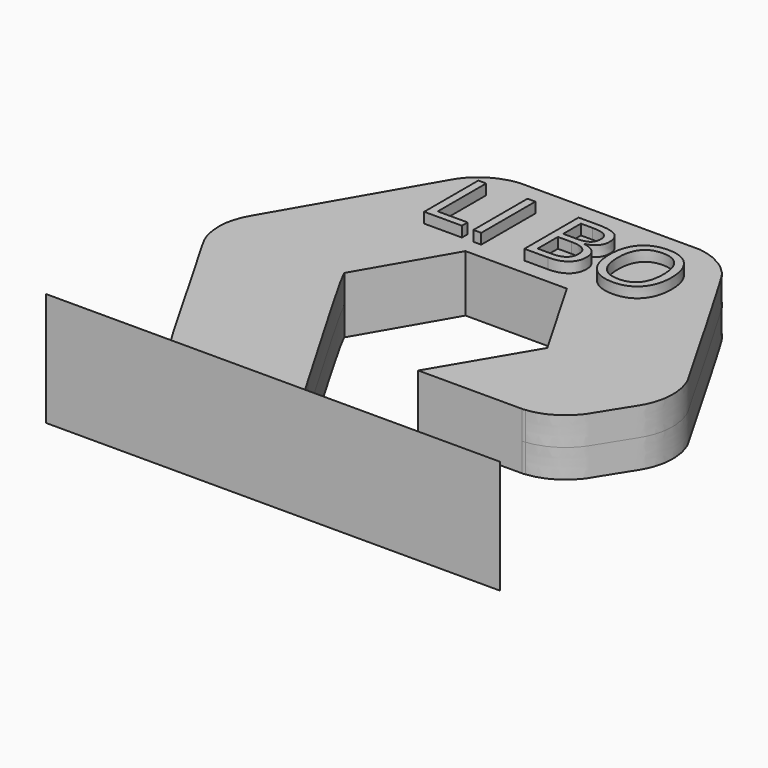
from build123d import *

# Parameters (mm, degrees)
F1_DEPTH     = 3.175
F2_DEPTH     = 1.5875
F3_DEPTH     = 1.5875
F4_T1_DEPTH  = 22.6801869736
F4_T3_DEPTH  = 41.7253830583
F5_TEXT_SIZE = 5.3007951162
F6_DEPTH     = 0.5842


# Not quite as in the source:
# - a fillet or chamfer that OpenCascade refuses, or shapes differently, is made with other operations: its cross-section is extruded or revolved along the edge and cut away or added
# - Text() gives the source's letters only with a copy of the font that has no kerning and outlines rounded to 1/6400 em; it was checked with that copy


with BuildPart() as f1:
    # F0 (on Top) → F1 (new body, symmetric)
    with BuildSketch(Plane.XY):
        with BuildLine():
            add(Edge.make_bspline(
                [(-8.0979492671, -8.4599665572), (-7.8144543772, -8.9512922446), (-7.4012331652, -9.6478596679), (-7.2094447017, -9.853233929), (-7.0198074368, -10.0624663427), (-6.8247908118, -10.2363901293), (-6.6355575508, -10.3900701529), (-6.4438841868, -10.5234739102), (-6.0350828964, -10.7264789939), (-5.8763022274, -10.78836422), (-5.4940772788, -10.9232334645), (-5.1611591338, -10.9716922009), (-4.9454318311, -10.9894729499), (-4.8368193396, -10.9980083466), (-1.8185705834, -10.9990381649), (0.9024133324, -10.9999665572)],
                knots=[0.5399683447, 0.5399683447, 0.5399683447, 0.5399683447, 0.583735527, 0.615598334, 0.6417416026, 0.6683965868, 0.6934366825, 0.7191935337, 0.7535274628, 0.7758085206, 0.8081226598, 0.8394404995, 0.861841058, 0.8754482187, 1, 1, 1, 1], degree=3))
            Line((-8.0979492671, -8.4599665572), (-12.7, -8.4599665572))
            Line((-12.7, -8.4599665572), (-12.7, -11.6349665572))
            Line((-12.7, -11.6349665572), (12.6951960847, -11.6349665572))
            Line((12.6951960847, -11.6349665572), (12.6951960847, -8.4599665572))
            Line((12.6951960847, -8.4599665572), (-0.5820742577, -8.4599665572))
            add(Edge.make_bspline(
                [(-0.5820742577, -8.4599665572), (-0.0948763272, -9.2939885426), (0.4037685026, -10.1469775499), (0.9024133324, -10.9999665572)],
                knots=[0.8523529488, 0.8523529488, 0.8523529488, 0.8523529488, 1, 1, 1, 1], degree=3))
        make_face()
        with BuildLine():
            Line((-0.5820742577, -8.4599665572), (-8.0979492671, -8.4599665572))
            add(Edge.make_bspline(
                [(-8.0979492671, -8.4599665572), (-7.8144543772, -8.9512922446), (-7.4012331652, -9.6478596679), (-7.2094447017, -9.853233929), (-7.0198074368, -10.0624663427), (-6.8247908118, -10.2363901293), (-6.6355575508, -10.3900701529), (-6.4438841868, -10.5234739102), (-6.0350828964, -10.7264789939), (-5.8763022274, -10.78836422), (-5.4940772788, -10.9232334645), (-5.1611591338, -10.9716922009), (-4.9454318311, -10.9894729499), (-4.8368193396, -10.9980083466), (-1.8185705834, -10.9990381649), (0.9024133324, -10.9999665572)],
                knots=[0.5399683447, 0.5399683447, 0.5399683447, 0.5399683447, 0.583735527, 0.615598334, 0.6417416026, 0.6683965868, 0.6934366825, 0.7191935337, 0.7535274628, 0.7758085206, 0.8081226598, 0.8394404995, 0.861841058, 0.8754482187, 1, 1, 1, 1], degree=3))
            add(Edge.make_bspline(
                [(-0.5820742577, -8.4599665572), (-0.0948763272, -9.2939885426), (0.4037685026, -10.1469775499), (0.9024133324, -10.9999665572)],
                knots=[0.8523529488, 0.8523529488, 0.8523529488, 0.8523529488, 1, 1, 1, 1], degree=3))
        make_face()
    extrude(amount=F1_DEPTH, both=True)

    # F0 (on Top) → F2 (cut, symmetric)
    with BuildSketch(Plane.XY):
        with BuildLine():
            add(Edge.make_bspline(
                [(-4.9467352219, 11.8727972619), (-2.6941970372, 11.8727972619), (-0.4416588525, 11.8727972619), (1.8108793323, 11.8727972619)],
                knots=[0.5524163134, 0.5524163134, 0.5524163134, 0.5524163134, 7.3100308676, 7.3100308676, 7.3100308676, 7.3100308676], degree=3))
            add(Edge.make_bspline(
                [(-12.1819954365, 2.2322773002), (-10.2153621206, 5.6292283823), (-7.918654142, 9.5963149713), (-7.7561059918, 9.8938723276), (-7.595936966, 10.1748103574), (-7.4488921306, 10.429639936), (-7.2380091716, 10.7143793357), (-7.0022497381, 10.9732635429), (-6.7468930063, 11.1814042046), (-6.6123462397, 11.2802086076), (-6.44534623, 11.390971666), (-6.3180815613, 11.463666659), (-6.1526142879, 11.5500745414), (-6.0434056072, 11.6051608595), (-5.8991320293, 11.660363592), (-5.6381957934, 11.7542790581), (-5.4211920209, 11.8110346891), (-5.1249038455, 11.8530818861), (-5.1009011539, 11.8676549492), (-4.9467352219, 11.8727972619)],
                knots=[0, 0, 0, 0, 0.1520022985, 0.1775139721, 0.2052814017, 0.2338919375, 0.2644870562, 0.2956347735, 0.3249719317, 0.3463123249, 0.3689682109, 0.3892301717, 0.411329997, 0.4293235674, 0.449497138, 0.4765503291, 0.5022012755, 0.5278147587, 0.5520405652, 0.5520405652, 0.5520405652, 0.5520405652], degree=3))
            add(Edge.make_bspline(
                [(-12.1819954365, 2.2322773002), (-12.2139037883, 2.1703194424), (-12.283482926, 2.0352145533), (-12.4406884255, 1.7801306072), (-12.6198918883, 1.2441500466), (-12.7164267868, 0.7551726738), (-12.7062312963, 0.3123164438), (-12.6510102494, -0.2863243011), (-12.5128439568, -0.6906531958), (-12.348735221, -1.0976190794), (-11.6470462247, -2.2552827891), (-11.0471565611, -3.3365181876), (-9.6670924889, -5.6885534643), (-8.4674528036, -7.819579074), (-8.0979492671, -8.4599665572)],
                knots=[0, 0, 0, 0, 0.0239021006, 0.0521207603, 0.0910959498, 0.1277402468, 0.1623042864, 0.2023672629, 0.23552051, 0.2695660314, 0.3281617082, 0.3861383143, 0.4829227709, 0.5399683447, 0.5399683447, 0.5399683447, 0.5399683447], degree=3))
            Line((-8.0979492671, -8.4599665572), (-0.5820742577, -8.4599665572))
            add(Edge.make_bspline(
                [(-5.6781647727, 0.4474149318), (-5.6798237666, 0.4432516249), (-5.716895521, 0.3502186819), (-3.2687593621, -3.8606973389), (-0.5820742577, -8.4599665572)],
                knots=[0, 0, 0, 0, 0.0381435521, 0.8523529488, 0.8523529488, 0.8523529488, 0.8523529488], degree=3))
            add(Edge.make_bspline(
                [(-2.836742904, 5.3628673777), (-3.7838835269, 3.7243832291), (-4.7310241498, 2.0858990805), (-5.6781647727, 0.4474149318)],
                knots=[0, 0, 0, 0, 5.6776184253, 5.6776184253, 5.6776184253, 5.6776184253], degree=3))
            add(Edge.make_bspline(
                [(2.8362337034, 5.3595150821), (0.9452415009, 5.360632514), (-0.9457507016, 5.3617499458), (-2.836742904, 5.3628673777)],
                knots=[0, 0, 0, 0, 5.6729775979, 5.6729775979, 5.6729775979, 5.6729775979], degree=3))
            add(Edge.make_bspline(
                [(5.6763379835, 0.4443899379), (4.7296365568, 2.082764986), (3.7829351301, 3.721140034), (2.8362337034, 5.3595150821)],
                knots=[0, 0, 0, 0, 5.6766757442, 5.6766757442, 5.6766757442, 5.6766757442], degree=3))
            add(Edge.make_bspline(
                [(2.6081528049, -4.7463672236), (3.6308811978, -3.0161148364), (4.6536095906, -1.2858624492), (5.6763379835, 0.4443899379)],
                knots=[0, 0, 0, 0, 6.0297363292, 6.0297363292, 6.0297363292, 6.0297363292], degree=3))
            Line((2.6081528049, -4.7463672236), (8.3983913064, -4.7463672236))
            add(Edge.make_bspline(
                [(8.3983913064, -4.7463672236), (8.4285802649, -4.7476342502), (8.4896773359, -4.7501984863), (8.5516653278, -4.7371940519), (8.5830241442, -4.7306152992)],
                knots=[0, 0, 0, 0, 0.4941146609, 1, 1, 1, 1], degree=3))
            add(Edge.make_bspline(
                [(7.394594606, 10.4755461216), (7.4049946498, 10.4644086633), (7.4978359113, 10.3649844979), (12.37583426, 1.9246802289), (12.3732313137, 1.8788009391), (12.4554314204, 1.7100351498), (12.5092309984, 1.5407375676), (12.579223391, 1.3481749221), (12.6327811924, 1.1548508933), (12.6617328431, 0.9474132467), (12.6887145756, 0.7331187902), (12.7057320419, 0.4773166934), (12.6885501549, 0.1892988959), (12.6579644324, -0.1503660031), (12.6047454763, -0.3551130001), (12.5476882015, -0.5689364186), (12.4644072913, -0.7996513773), (12.3592844301, -1.0395808564), (12.2025247276, -1.3122675142), (11.5798542764, -2.2842021351), (11.0022863487, -3.2119016224), (10.8931559285, -3.3988812592), (10.7117863794, -3.6224692911), (10.497630846, -3.8442513774), (10.2817003921, -4.0291717223), (10.0560553294, -4.2067210739), (9.8433649464, -4.3187164368), (9.7865197525, -4.3546553415), (9.5130416542, -4.505924573), (9.2077822138, -4.5905623978), (9.0144989656, -4.6706733119), (8.6495598585, -4.7218623963), (8.5981329416, -4.7286277074), (8.5830241442, -4.7306152992)],
                knots=[0, 0, 0, 0, 0.0211617068, 0.1889107002, 0.2086954298, 0.2296465529, 0.2530764843, 0.2773859957, 0.3015816681, 0.3261482383, 0.3512044462, 0.3783001026, 0.40768826, 0.4390979831, 0.4639315394, 0.4889953709, 0.5158573886, 0.5426802508, 0.5721507083, 0.6312181763, 0.6877344447, 0.7121562897, 0.7402266081, 0.7704940169, 0.7992541414, 0.828820597, 0.8543275782, 0.8684516809, 0.8979328023, 0.9286239977, 0.9544581079, 0.9866201736, 1, 1, 1, 1], degree=3))
            add(Edge.make_bspline(
                [(5.0841737539, 11.8727972619), (5.1354007842, 11.8660248609), (5.285102127, 11.8344246259), (5.511192311, 11.7972110307), (5.856974007, 11.6822825291), (6.0571511062, 11.6028524692), (6.5572225021, 11.3301125557), (6.8102335511, 11.1329565648), (7.0714115659, 10.8810767284), (7.2647332021, 10.6836819238), (7.3523685742, 10.5432240362), (7.394594606, 10.4755461216)],
                knots=[0.7441231562, 0.7441231562, 0.7441231562, 0.7441231562, 0.7668331465, 0.7924407066, 0.8229285687, 0.8479598314, 0.8863005426, 0.9166541286, 0.9473218688, 0.974617687, 1, 1, 1, 1], degree=3))
            add(Edge.make_bspline(
                [(4.7206622548, 11.8727972619), (4.8418327545, 11.8727972619), (4.9630032542, 11.8727972619), (5.0841737539, 11.8727972619)],
                knots=[10.2198137902, 10.2198137902, 10.2198137902, 10.2198137902, 10.5833252892, 10.5833252892, 10.5833252892, 10.5833252892], degree=3))
            add(Edge.make_bspline(
                [(1.8108793323, 11.8727972619), (3.1458171486, 11.8689304093), (4.2714307431, 11.8669693291), (4.7206622548, 11.8727972619)],
                knots=[0.6587883417, 0.6587883417, 0.6587883417, 0.6587883417, 0.7129256384, 0.7129256384, 0.7129256384, 0.7129256384], degree=3))
        make_face()
        with BuildLine():
            Line((-0.5820742577, -8.4599665572), (-8.0979492671, -8.4599665572))
            add(Edge.make_bspline(
                [(-8.0979492671, -8.4599665572), (-7.8144543772, -8.9512922446), (-7.4012331652, -9.6478596679), (-7.2094447017, -9.853233929), (-7.0198074368, -10.0624663427), (-6.8247908118, -10.2363901293), (-6.6355575508, -10.3900701529), (-6.4438841868, -10.5234739102), (-6.0350828964, -10.7264789939), (-5.8763022274, -10.78836422), (-5.4940772788, -10.9232334645), (-5.1611591338, -10.9716922009), (-4.9454318311, -10.9894729499), (-4.8368193396, -10.9980083466), (-1.8185705834, -10.9990381649), (0.9024133324, -10.9999665572)],
                knots=[0.5399683447, 0.5399683447, 0.5399683447, 0.5399683447, 0.583735527, 0.615598334, 0.6417416026, 0.6683965868, 0.6934366825, 0.7191935337, 0.7535274628, 0.7758085206, 0.8081226598, 0.8394404995, 0.861841058, 0.8754482187, 1, 1, 1, 1], degree=3))
            add(Edge.make_bspline(
                [(-0.5820742577, -8.4599665572), (-0.0948763272, -9.2939885426), (0.4037685026, -10.1469775499), (0.9024133324, -10.9999665572)],
                knots=[0.8523529488, 0.8523529488, 0.8523529488, 0.8523529488, 1, 1, 1, 1], degree=3))
        make_face()
    extrude(amount=F2_DEPTH, both=True, mode=Mode.SUBTRACT)

    # F4: chamfer of 3.175 on 4 edges, made by hand

    # F4_s2 → F4_t1 (cut)
    with BuildSketch(Plane.XY.offset(-11.3400934868)):
        Polygon((-9.525, -8.4599665572), (-12.7, -11.6349665572), (-12.7, -8.4599665572), align=None)
        Polygon((9.5201960847, -8.4599665572), (12.6951960847, -11.6349665572), (12.6951960847, -8.4599665572), align=None)
    extrude(amount=F4_T1_DEPTH, mode=Mode.SUBTRACT)

    # F4_s4 → F4_t3 (cut)
    with BuildSketch(Plane.YZ.offset(-20.8650934868)):
        Polygon((-8.4599665572, 0), (-11.6349665572, 3.175), (-8.4599665572, 3.175), align=None)
        Polygon((-8.4599665572, 0), (-11.6349665572, -3.175), (-8.4599665572, -3.175), align=None)
    extrude(amount=F4_T3_DEPTH, mode=Mode.SUBTRACT)


with BuildPart() as f3:
    # F0 (on Top) → F3 (new body, symmetric)
    with BuildSketch(Plane.XY):
        with BuildLine():
            add(Edge.make_bspline(
                [(-4.9467352219, 11.8727972619), (-2.6941970372, 11.8727972619), (-0.4416588525, 11.8727972619), (1.8108793323, 11.8727972619)],
                knots=[0.5524163134, 0.5524163134, 0.5524163134, 0.5524163134, 7.3100308676, 7.3100308676, 7.3100308676, 7.3100308676], degree=3))
            add(Edge.make_bspline(
                [(-12.1819954365, 2.2322773002), (-10.2153621206, 5.6292283823), (-7.918654142, 9.5963149713), (-7.7561059918, 9.8938723276), (-7.595936966, 10.1748103574), (-7.4488921306, 10.429639936), (-7.2380091716, 10.7143793357), (-7.0022497381, 10.9732635429), (-6.7468930063, 11.1814042046), (-6.6123462397, 11.2802086076), (-6.44534623, 11.390971666), (-6.3180815613, 11.463666659), (-6.1526142879, 11.5500745414), (-6.0434056072, 11.6051608595), (-5.8991320293, 11.660363592), (-5.6381957934, 11.7542790581), (-5.4211920209, 11.8110346891), (-5.1249038455, 11.8530818861), (-5.1009011539, 11.8676549492), (-4.9467352219, 11.8727972619)],
                knots=[0, 0, 0, 0, 0.1520022985, 0.1775139721, 0.2052814017, 0.2338919375, 0.2644870562, 0.2956347735, 0.3249719317, 0.3463123249, 0.3689682109, 0.3892301717, 0.411329997, 0.4293235674, 0.449497138, 0.4765503291, 0.5022012755, 0.5278147587, 0.5520405652, 0.5520405652, 0.5520405652, 0.5520405652], degree=3))
            add(Edge.make_bspline(
                [(-12.1819954365, 2.2322773002), (-12.2139037883, 2.1703194424), (-12.283482926, 2.0352145533), (-12.4406884255, 1.7801306072), (-12.6198918883, 1.2441500466), (-12.7164267868, 0.7551726738), (-12.7062312963, 0.3123164438), (-12.6510102494, -0.2863243011), (-12.5128439568, -0.6906531958), (-12.348735221, -1.0976190794), (-11.6470462247, -2.2552827891), (-11.0471565611, -3.3365181876), (-9.6670924889, -5.6885534643), (-8.4674528036, -7.819579074), (-8.0979492671, -8.4599665572)],
                knots=[0, 0, 0, 0, 0.0239021006, 0.0521207603, 0.0910959498, 0.1277402468, 0.1623042864, 0.2023672629, 0.23552051, 0.2695660314, 0.3281617082, 0.3861383143, 0.4829227709, 0.5399683447, 0.5399683447, 0.5399683447, 0.5399683447], degree=3))
            Line((-8.0979492671, -8.4599665572), (-0.5820742577, -8.4599665572))
            add(Edge.make_bspline(
                [(-5.6781647727, 0.4474149318), (-5.6798237666, 0.4432516249), (-5.716895521, 0.3502186819), (-3.2687593621, -3.8606973389), (-0.5820742577, -8.4599665572)],
                knots=[0, 0, 0, 0, 0.0381435521, 0.8523529488, 0.8523529488, 0.8523529488, 0.8523529488], degree=3))
            add(Edge.make_bspline(
                [(-2.836742904, 5.3628673777), (-3.7838835269, 3.7243832291), (-4.7310241498, 2.0858990805), (-5.6781647727, 0.4474149318)],
                knots=[0, 0, 0, 0, 5.6776184253, 5.6776184253, 5.6776184253, 5.6776184253], degree=3))
            add(Edge.make_bspline(
                [(2.8362337034, 5.3595150821), (0.9452415009, 5.360632514), (-0.9457507016, 5.3617499458), (-2.836742904, 5.3628673777)],
                knots=[0, 0, 0, 0, 5.6729775979, 5.6729775979, 5.6729775979, 5.6729775979], degree=3))
            add(Edge.make_bspline(
                [(5.6763379835, 0.4443899379), (4.7296365568, 2.082764986), (3.7829351301, 3.721140034), (2.8362337034, 5.3595150821)],
                knots=[0, 0, 0, 0, 5.6766757442, 5.6766757442, 5.6766757442, 5.6766757442], degree=3))
            add(Edge.make_bspline(
                [(2.6081528049, -4.7463672236), (3.6308811978, -3.0161148364), (4.6536095906, -1.2858624492), (5.6763379835, 0.4443899379)],
                knots=[0, 0, 0, 0, 6.0297363292, 6.0297363292, 6.0297363292, 6.0297363292], degree=3))
            Line((2.6081528049, -4.7463672236), (8.3983913064, -4.7463672236))
            add(Edge.make_bspline(
                [(8.3983913064, -4.7463672236), (8.4285802649, -4.7476342502), (8.4896773359, -4.7501984863), (8.5516653278, -4.7371940519), (8.5830241442, -4.7306152992)],
                knots=[0, 0, 0, 0, 0.4941146609, 1, 1, 1, 1], degree=3))
            add(Edge.make_bspline(
                [(7.394594606, 10.4755461216), (7.4049946498, 10.4644086633), (7.4978359113, 10.3649844979), (12.37583426, 1.9246802289), (12.3732313137, 1.8788009391), (12.4554314204, 1.7100351498), (12.5092309984, 1.5407375676), (12.579223391, 1.3481749221), (12.6327811924, 1.1548508933), (12.6617328431, 0.9474132467), (12.6887145756, 0.7331187902), (12.7057320419, 0.4773166934), (12.6885501549, 0.1892988959), (12.6579644324, -0.1503660031), (12.6047454763, -0.3551130001), (12.5476882015, -0.5689364186), (12.4644072913, -0.7996513773), (12.3592844301, -1.0395808564), (12.2025247276, -1.3122675142), (11.5798542764, -2.2842021351), (11.0022863487, -3.2119016224), (10.8931559285, -3.3988812592), (10.7117863794, -3.6224692911), (10.497630846, -3.8442513774), (10.2817003921, -4.0291717223), (10.0560553294, -4.2067210739), (9.8433649464, -4.3187164368), (9.7865197525, -4.3546553415), (9.5130416542, -4.505924573), (9.2077822138, -4.5905623978), (9.0144989656, -4.6706733119), (8.6495598585, -4.7218623963), (8.5981329416, -4.7286277074), (8.5830241442, -4.7306152992)],
                knots=[0, 0, 0, 0, 0.0211617068, 0.1889107002, 0.2086954298, 0.2296465529, 0.2530764843, 0.2773859957, 0.3015816681, 0.3261482383, 0.3512044462, 0.3783001026, 0.40768826, 0.4390979831, 0.4639315394, 0.4889953709, 0.5158573886, 0.5426802508, 0.5721507083, 0.6312181763, 0.6877344447, 0.7121562897, 0.7402266081, 0.7704940169, 0.7992541414, 0.828820597, 0.8543275782, 0.8684516809, 0.8979328023, 0.9286239977, 0.9544581079, 0.9866201736, 1, 1, 1, 1], degree=3))
            add(Edge.make_bspline(
                [(5.0841737539, 11.8727972619), (5.1354007842, 11.8660248609), (5.285102127, 11.8344246259), (5.511192311, 11.7972110307), (5.856974007, 11.6822825291), (6.0571511062, 11.6028524692), (6.5572225021, 11.3301125557), (6.8102335511, 11.1329565648), (7.0714115659, 10.8810767284), (7.2647332021, 10.6836819238), (7.3523685742, 10.5432240362), (7.394594606, 10.4755461216)],
                knots=[0.7441231562, 0.7441231562, 0.7441231562, 0.7441231562, 0.7668331465, 0.7924407066, 0.8229285687, 0.8479598314, 0.8863005426, 0.9166541286, 0.9473218688, 0.974617687, 1, 1, 1, 1], degree=3))
            add(Edge.make_bspline(
                [(4.7206622548, 11.8727972619), (4.8418327545, 11.8727972619), (4.9630032542, 11.8727972619), (5.0841737539, 11.8727972619)],
                knots=[10.2198137902, 10.2198137902, 10.2198137902, 10.2198137902, 10.5833252892, 10.5833252892, 10.5833252892, 10.5833252892], degree=3))
            add(Edge.make_bspline(
                [(1.8108793323, 11.8727972619), (3.1458171486, 11.8689304093), (4.2714307431, 11.8669693291), (4.7206622548, 11.8727972619)],
                knots=[0.6587883417, 0.6587883417, 0.6587883417, 0.6587883417, 0.7129256384, 0.7129256384, 0.7129256384, 0.7129256384], degree=3))
        make_face()
        with BuildLine():
            Line((-0.5820742577, -8.4599665572), (-8.0979492671, -8.4599665572))
            add(Edge.make_bspline(
                [(-8.0979492671, -8.4599665572), (-7.8144543772, -8.9512922446), (-7.4012331652, -9.6478596679), (-7.2094447017, -9.853233929), (-7.0198074368, -10.0624663427), (-6.8247908118, -10.2363901293), (-6.6355575508, -10.3900701529), (-6.4438841868, -10.5234739102), (-6.0350828964, -10.7264789939), (-5.8763022274, -10.78836422), (-5.4940772788, -10.9232334645), (-5.1611591338, -10.9716922009), (-4.9454318311, -10.9894729499), (-4.8368193396, -10.9980083466), (-1.8185705834, -10.9990381649), (0.9024133324, -10.9999665572)],
                knots=[0.5399683447, 0.5399683447, 0.5399683447, 0.5399683447, 0.583735527, 0.615598334, 0.6417416026, 0.6683965868, 0.6934366825, 0.7191935337, 0.7535274628, 0.7758085206, 0.8081226598, 0.8394404995, 0.861841058, 0.8754482187, 1, 1, 1, 1], degree=3))
            add(Edge.make_bspline(
                [(-0.5820742577, -8.4599665572), (-0.0948763272, -9.2939885426), (0.4037685026, -10.1469775499), (0.9024133324, -10.9999665572)],
                knots=[0.8523529488, 0.8523529488, 0.8523529488, 0.8523529488, 1, 1, 1, 1], degree=3))
        make_face()
    extrude(amount=F3_DEPTH, both=True)

    # F5 (on face) → F6 (join)
    with BuildSketch(Plane.XY.offset(1.5875)):
        with Locations((-6.3892700709, 6.2664556317)):
            Text('LI BO', F5_TEXT_SIZE, font='Open Sans', text_align=(TextAlign.LEFT, TextAlign.BOTTOM))
    extrude(amount=F6_DEPTH)


solid = Compound([f1.part, f3.part])
